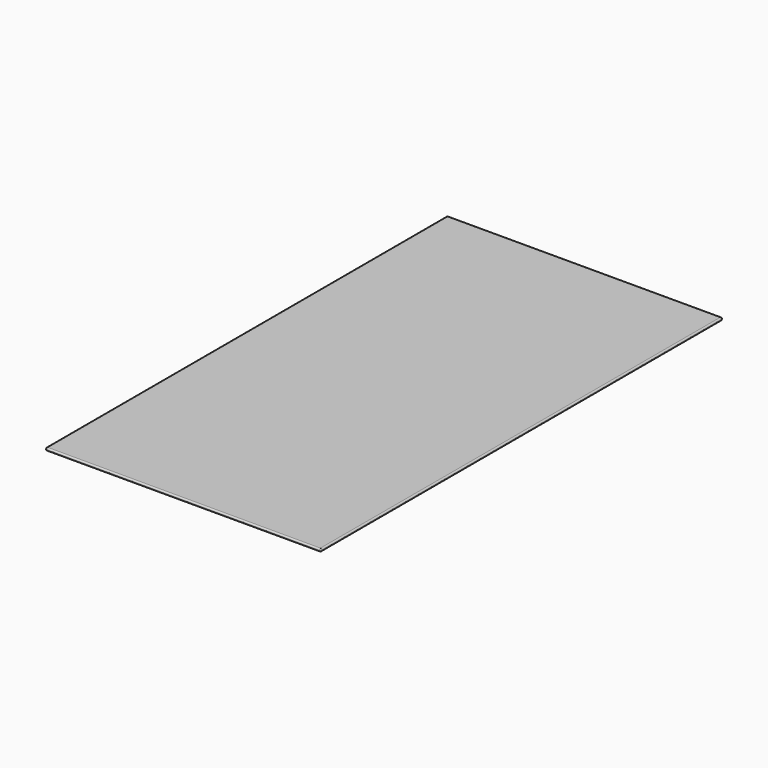
from build123d import *

# Parameters (mm, degrees)
F0_W     = 100.076
F0_H     = 182.626
F1_DEPTH = 1.016
F2_R     = 0.50799


# Not quite as in the source:
# - a fillet or chamfer is up to 0.001 mm smaller than in the source, because OpenCascade refuses the exact size


with BuildPart() as f1:
    # F0 (on Top) → F1 (new body)
    with BuildSketch(Plane.XY):
        Rectangle(F0_W, F0_H)
    extrude(amount=F1_DEPTH)

    # F2 (radius 0.508 in the source; OpenCascade refuses exactly that, so slightly less here)
    f2_edges = [f1.edges().sort_by_distance(p)[0] for p in [
        (50.038, -91.313, 0.508),
        (50.038, 91.313, 0.508),
        (50.038, 0, 0),
        (50.038, 0, 1.016),
        (-50.038, -91.313, 0.508),
        (0, -91.313, 0),
        (0, -91.313, 1.016),
        (-50.038, 91.313, 0.508),
        (-50.038, 0, 0),
        (-50.038, 0, 1.016),
        (0, 91.313, 0),
        (0, 91.313, 1.016),
    ]]
    fillet(f2_edges, radius=F2_R)


solid = f1.part
